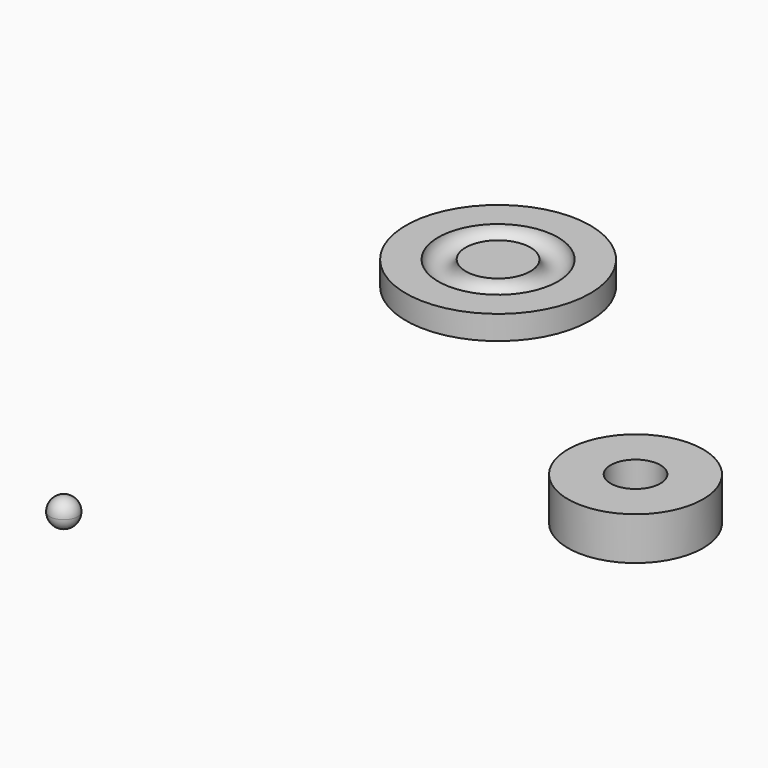
from build123d import *

# Parameters (mm, degrees)
F0_R      = 11
F0_R_2    = 2.5
F1_DEPTH  = 7
F2_R      = 2.25
F3_DEPTH  = 4.5
F4_R      = 2.24999
F5_R      = 15
F6_DEPTH  = 3.9
F11_R     = 4.05
F12_DEPTH = 25


# Not quite as in the source:
# - a fillet or chamfer is up to 0.001 mm smaller than in the source, because OpenCascade refuses the exact size


with BuildPart() as f1:
    # F0 (on Top) → F1 (new body)
    with BuildSketch(Plane.XY):
        Circle(F0_R)
        Circle(F0_R_2, mode=Mode.SUBTRACT)
    extrude(amount=F1_DEPTH)

    # F11 (on face) → F12 (cut)
    with BuildSketch(Plane.XY.offset(7)):
        Circle(F11_R)
    extrude(amount=-F12_DEPTH, mode=Mode.SUBTRACT)


with BuildPart() as f3:
    # F2 (on Top) → F3 (new body)
    with BuildSketch(Plane.XY):
        with Locations((-56.030407548, -46.2823361158)):
            Circle(F2_R)
    extrude(amount=F3_DEPTH)

    # F4 (radius 2.25 in the source; OpenCascade refuses exactly that, so slightly less here)
    f4_edges = [f3.edges().sort_by_distance(p)[0] for p in [
        (-58.280408, -46.282336, 4.5),
        (-58.280408, -46.282336, 0),
    ]]
    fillet(f4_edges, radius=F4_R)


with BuildPart() as f6:
    # F5 (on Top) → F6 (new body)
    with BuildSketch(Plane.XY):
        with Locations((-54.3050132692, 39.9165041745)):
            Circle(F5_R)
    extrude(amount=F6_DEPTH)

    # F9 (on line) → F10 (revolve, cut)
    with BuildSketch(Plane(origin=(0, 39.9165041745, 0), x_dir=(-1, 0, 0), z_dir=(0, 1, 0))):
        with BuildLine():
            Line((49.0550132692, 4.15), (44.5550132692, 4.15))
            ThreePointArc((44.5550132692, 4.15), (46.8050132692, 1.9), (49.0550132692, 4.15))
        make_face()
    revolve(axis=Axis((-54.3050132692, 39.9165041745, 3.9), (0, 0, 1)), mode=Mode.SUBTRACT)


solid = Compound([f1.part, f3.part, f6.part])
